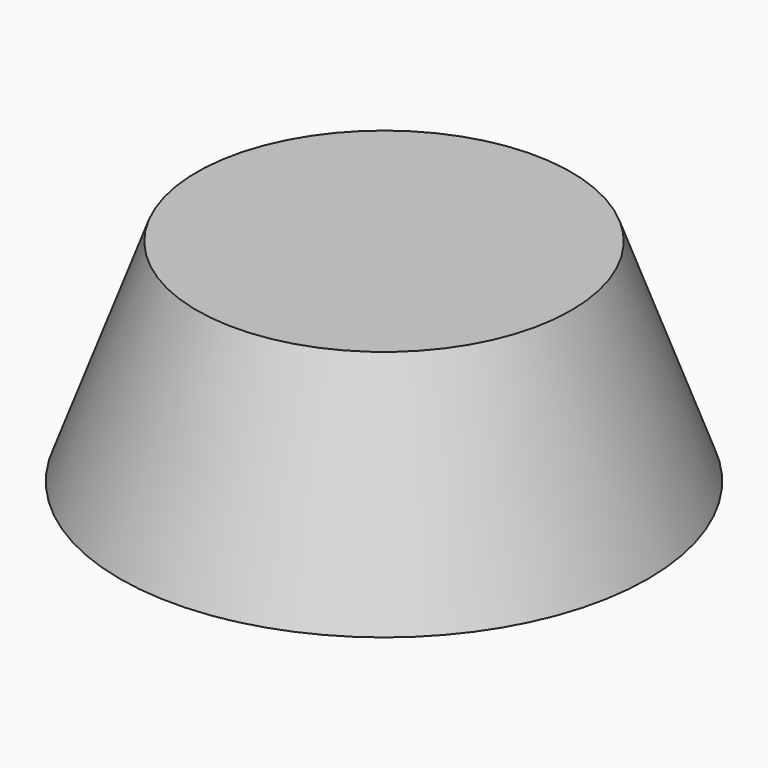
from build123d import *

# Parameters (mm, degrees)
F0_R     = 125
F1_DEPTH = 100
F2_SIZE2 = 36.397013
F2_SIZE  = 99.99999


# Not quite as in the source:
# - a fillet or chamfer is up to 0.001 mm smaller than in the source, because OpenCascade refuses the exact size


with BuildPart() as f1:
    # F0 (on Top) → F1 (new body)
    with BuildSketch(Plane.XY):
        Circle(F0_R)
    extrude(amount=F1_DEPTH)

    # F2 (size 100 and 36.3970234266 in the source; OpenCascade refuses exactly that, so slightly less here)
    f2_edges = [f1.edges().sort_by_distance(p)[0] for p in [
        (-125, 0, 100),
    ]]
    f2_side = f1.faces().sort_by_distance((-125, 0, 50))[0]
    chamfer(f2_edges, length=F2_SIZE, length2=F2_SIZE2, reference=f2_side)


solid = f1.part
